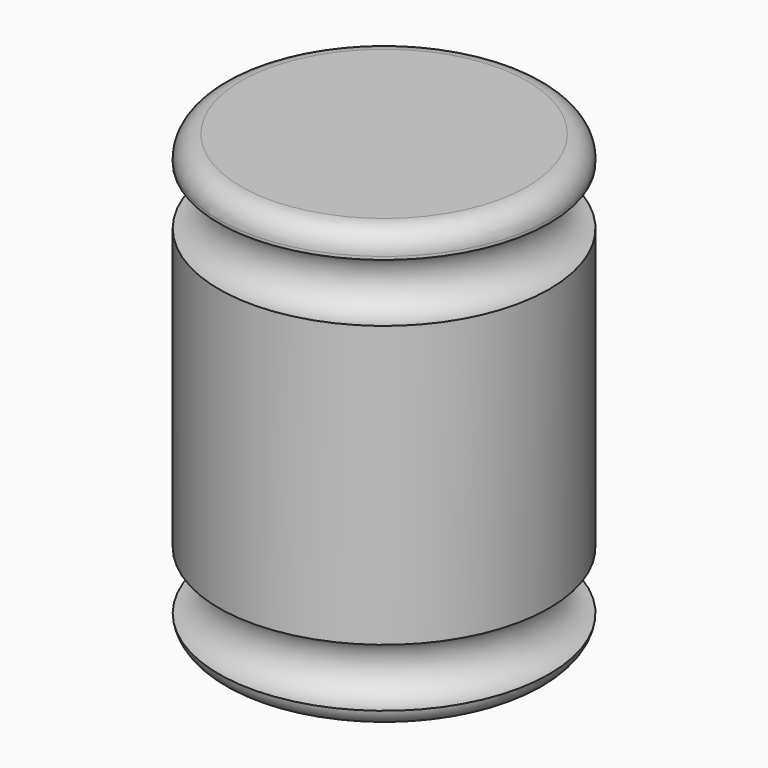
from build123d import *


# Not quite as in the source:
# - a fillet or chamfer that OpenCascade refuses, or shapes differently, is made with other operations: its cross-section is extruded or revolved along the edge and cut away or added


with BuildPart() as f1:
    # F0 (on Front) → F1 (revolve)
    with BuildSketch(Plane.XZ):
        with BuildLine():
            Line((-38.1, 0), (0, 0))
            Line((0, 0), (0, 4.2121557752))
            ThreePointArc((0, 4.2121557752), (-6.7056, 10.9177557752), (0, 17.6233557752))
            Line((0, 17.6233557752), (0, 82.4117260776))
            ThreePointArc((0, 82.4117260776), (-6.7019564309, 89.1136825085), (0, 95.8156389394))
            Line((0, 95.8156389394), (0, 101.6))
            Line((0, 101.6), (-38.1, 101.6))
            Line((-38.1, 101.6), (-38.1, 0))
        make_face()
    revolve(axis=Axis((-38.1, 0, 50.8), (0, 0, 1)))

    # F2: fillet of radius 5.08 on 2 edges, made by hand

    # F2_s1 → F2_t2 (revolve, cut)
    with BuildSketch(Plane.XZ):
        with BuildLine():
            ThreePointArc((0, 96.52), (-1.4878975516, 100.1121024484), (-5.08, 101.6))
            Line((-5.08, 101.6), (0, 101.6))
            Line((0, 101.6), (0, 96.52))
        make_face()
    revolve(axis=Axis((-38.1, 0, 101.6), (0, 0, 1)), mode=Mode.SUBTRACT)

    # F2_s3 → F2_t4 (revolve, cut)
    with BuildSketch(Plane.XZ):
        with BuildLine():
            ThreePointArc((-5.005321808, 0), (-1.7344082248, 1.1931601099), (0, 4.2121557752))
            Line((0, 4.2121557752), (0, 0))
            Line((0, 0), (-5.005321808, 0))
        make_face()
    revolve(axis=Axis((-38.1, 0, 0), (0, 0, 1)), mode=Mode.SUBTRACT)


solid = f1.part
